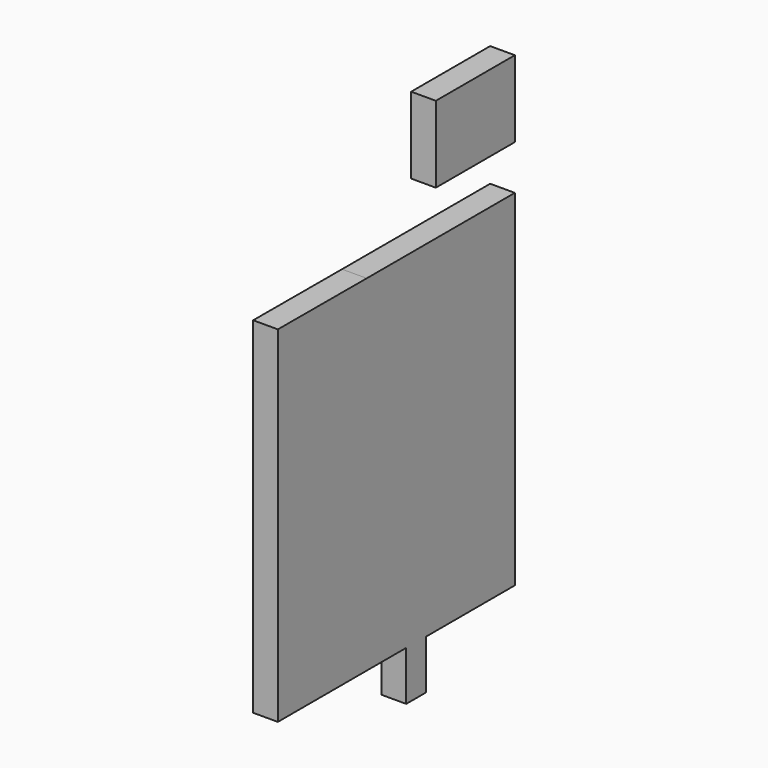
from build123d import *

# Parameters (mm, degrees)
F1_DEPTH = 5


# Not quite as in the source:
# - a feature names something its author has since deleted; it is built from what else it names


with BuildPart() as f1:
    # F0 (on Right) → F1 (new body)
    with BuildSketch(Plane.YZ):
        Polygon((22.5, -0.0434386059), (0, 0), (0, -70), (12, -70), (12.4011761725, -70), (32.5, -70), (32.5, -80), (37.5, -80), (37.5, -70.0434386059), (60, -70.0434386059), (60, -0.0434386059), align=None)
    extrude(amount=F1_DEPTH)


with BuildPart() as f1b:
    # F0 (on Right) → F1, piece 2 (new body)
    with BuildSketch(Plane.YZ):
        Polygon((40, 8.9999613941), (42.5, 8.9999613941), (60, 8.9999613941), (60, 24.499980697), (42.5, 24.499980697), (40, 24.499980697), align=None)
    extrude(amount=F1_DEPTH)


solid = Compound([f1.part, f1b.part])
